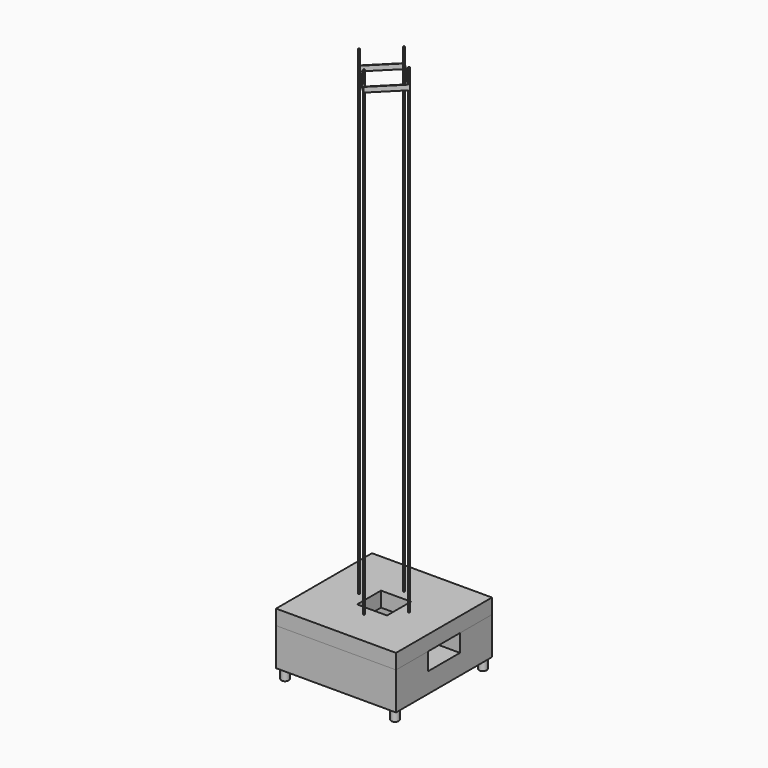
from build123d import *

# Parameters (mm, degrees)
F1_DEPTH  = 38.1
F3_DEPTH  = 152.4
F5_DEPTH  = 44.45
F6_R      = 9.525
F7_DEPTH  = 25.4
F8_R      = 1.5875
F9_DEPTH  = 1219.2
F12_DEPTH = 12.7


with BuildPart() as f1:
    # F0 (on Top) → F1 (new body)
    with BuildSketch(Plane.XY):
        Polygon((-152.4, 152.4), (-152.4, 0), (-152.4, -152.4), (152.4, -152.4), (152.4, 0), (152.4, 152.4), align=None)
        Polygon((-38.1, 38.1), (0, 38.1), (38.1, 38.1), (38.1, -38.1), (-38.1, -38.1), align=None, mode=Mode.SUBTRACT)
    extrude(amount=F1_DEPTH)

    # F8 (on face) → F9 (join)
    with BuildSketch(Plane.XY.offset(38.1)):
        with Locations((0, 63.5)):
            Circle(F8_R)
        with Locations((63.5, 0)):
            Circle(F8_R)
        with Locations((-63.5, 0)):
            Circle(F8_R)
        with Locations((0, -63.5)):
            Circle(F8_R)
    extrude(amount=F9_DEPTH)

    # F11 (on offset) → F12 (join)
    with BuildSketch(Plane(origin=(0, 0, 1219.2), x_dir=(1, 0, 0), z_dir=(0, 0, -1))):
        Polygon((0, -65.7450640303), (1.1225320151, -64.6225320151), (64.6225320151, -1.1225320151), (65.7450640303, 0), (1.1225320151, 64.6225320151), (0, 65.7450640303), (-65.7450640303, 0), (-64.6225320151, -1.1225320151), align=None)
        Polygon((0, -63.5), (-63.5, 0), (0, 63.5), (63.5, 0), align=None, mode=Mode.SUBTRACT)
    extrude(amount=F12_DEPTH)


with BuildPart() as f3:
    # F2 (on Front) → F3 (new body, symmetric)
    with BuildSketch(Plane.XZ):
        with BuildLine():
            ThreePointArc((31.75, -44.45), (13.2229437572, -35.0650703036), (0, -19.05))
            Line((0, -19.05), (0, -44.45))
            Line((0, -44.45), (31.75, -44.45))
        make_face()
        with BuildLine():
            Line((0, -44.45), (0, -19.05))
            ThreePointArc((0, -19.05), (-13.2229437572, -35.0650703036), (-31.75, -44.45))
            Line((-31.75, -44.45), (0, -44.45))
        make_face()
        Polygon((31.75, -44.45), (0, -44.45), (-31.75, -44.45), (-152.4, -44.45), (-152.4, -95.25), (152.4, -95.25), (152.4, -44.45), align=None)
    extrude(amount=F3_DEPTH, both=True)

    # F4 (on face) → F5 (join)
    with BuildSketch(Plane.XY.offset(-44.45)):
        Polygon((152.4, -50.8), (0, -50.8), (-152.4, -50.8), (-152.4, -152.4), (152.4, -152.4), align=None)
        Polygon((-152.4, 50.8), (0, 50.8), (152.4, 50.8), (152.4, 152.4), (-152.4, 152.4), align=None)
    extrude(amount=F5_DEPTH)

    # F6 (on face) → F7 (join)
    with BuildSketch(Plane(origin=(0, 0, -95.25), x_dir=(1, 0, 0), z_dir=(0, 0, -1))):
        with Locations((-139.7, 139.7)):
            Circle(F6_R)
        with Locations((139.7, 139.7)):
            Circle(F6_R)
        with Locations((139.7, -139.7)):
            Circle(F6_R)
        with Locations((-139.7, -139.7)):
            Circle(F6_R)
        Circle(F6_R)
    extrude(amount=F7_DEPTH)


solid = Compound([f1.part, f3.part])
